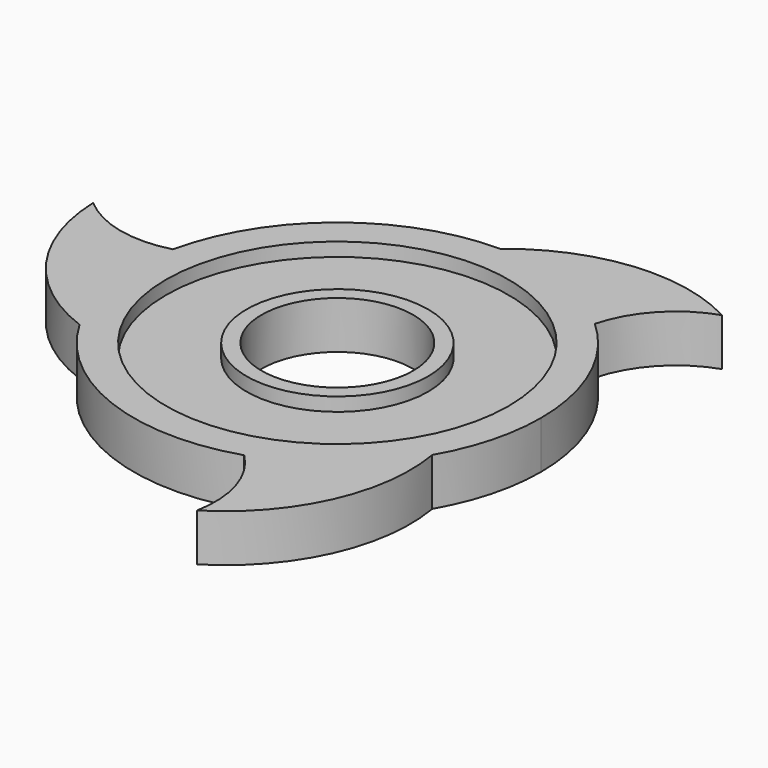
from build123d import *

# Parameters (mm, degrees)
F0_R     = 13.3742316953
F0_R_2   = 11.165
F1_DEPTH = 7
F0_R_3   = 25.2344394366
F2_DEPTH = 5
F3_DEPTH = 2


with BuildPart() as f1:
    # F0 (on Top) → F1 (new body)
    with BuildSketch(Plane.XY):
        Circle(F0_R)
        Circle(F0_R_2, mode=Mode.SUBTRACT)
    extrude(amount=F1_DEPTH)


with BuildPart() as f1b:
    # F0 (on Top) → F1, piece 2 (new body)
    with BuildSketch(Plane.XY):
        with BuildLine():
            ThreePointArc((25.9807621135, -15), (28.9777747887, -7.7645713531), (30, 0))
            ThreePointArc((30, 0), (27.4350087398, 12.1375572273), (20.1786469702, 22.1995992408))
            ThreePointArc((20.1786469702, 22.1995992408), (10.8169316993, 27.9820297443), (0, 30))
            ThreePointArc((0, 30), (-18.8246827584, 23.3587525148), (-29.3147403815, 6.3754212698))
            ThreePointArc((-29.3147403815, 6.3754212698), (-29.6416144577, -4.6232772295), (-25.9807621135, -15))
            ThreePointArc((-25.9807621135, -15), (-10.8169316993, -27.9820297443), (9.1360934113, -28.5750205106))
            ThreePointArc((9.1360934113, -28.5750205106), (18.8246827584, -23.3587525148), (25.9807621135, -15))
        make_face()
        Circle(F0_R_3, mode=Mode.SUBTRACT)
        with BuildLine():
            ThreePointArc((0, 30), (10.8169316993, 27.9820297443), (20.1786469702, 22.1995992408))
            ThreePointArc((20.1786469702, 22.1995992408), (23.849043869, 28.8770888286), (30.2408803254, 33.0249927938))
            ThreePointArc((30.2408803254, 33.0249927938), (14.6589394966, 36.1261227315), (0, 30))
        make_face()
        with BuildLine():
            ThreePointArc((-25.9807621135, -15), (-29.6416144577, -4.6232772295), (-29.3147403815, 6.3754212698))
            ThreePointArc((-29.3147403815, 6.3754212698), (-36.9328144474, 6.2153334322), (-43.7209228819, 9.6768741977))
            ThreePointArc((-43.7209228819, 9.6768741977), (-38.615609774, -5.3680473692), (-25.9807621135, -15))
        make_face()
        with BuildLine():
            ThreePointArc((13.4800425565, -42.7018669915), (23.9566702775, -30.7580753623), (25.9807621135, -15))
            ThreePointArc((25.9807621135, -15), (18.8246827584, -23.3587525148), (9.1360934113, -28.5750205106))
            ThreePointArc((9.1360934113, -28.5750205106), (13.0837705784, -35.0924222608), (13.4800425565, -42.7018669915))
        make_face()
    extrude(amount=F1_DEPTH)


with BuildPart() as f2:
    # F0 (on Top) → F2 (new body)
    with BuildSketch(Plane.XY):
        Circle(F0_R_3)
        Circle(F0_R, mode=Mode.SUBTRACT)
    extrude(amount=F2_DEPTH)

    # F0 (on Top) → F3 (cut)
    with BuildSketch(Plane.XY):
        Circle(F0_R_3)
        Circle(F0_R, mode=Mode.SUBTRACT)
    extrude(amount=F3_DEPTH, mode=Mode.SUBTRACT)


solid = Compound([f1.part, f1b.part, f2.part])
